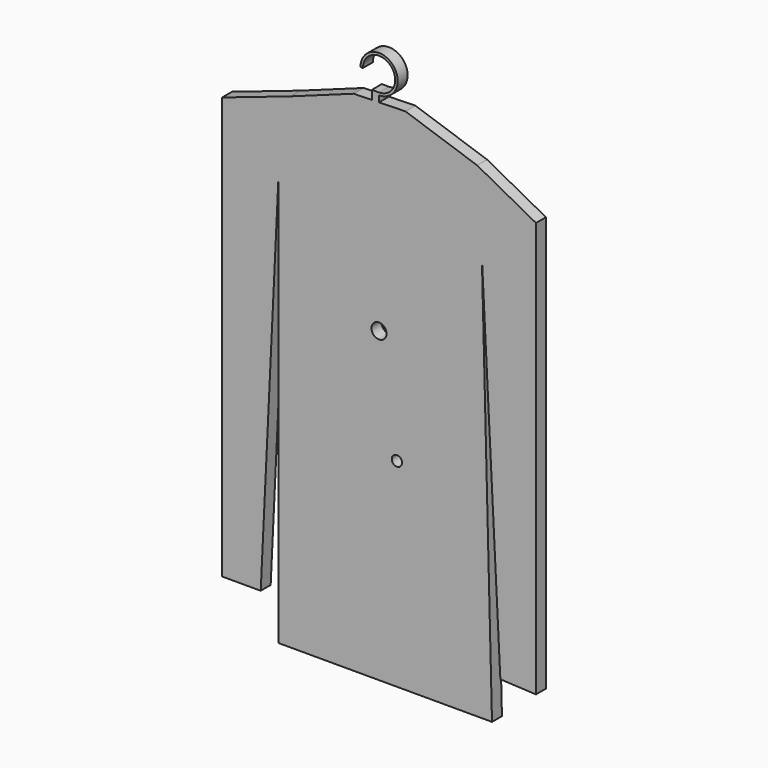
from build123d import *

# Parameters (mm, degrees)
F0_R     = 10.3520416824
F0_R_2   = 15.1016918028
F1_DEPTH = 12.5


with BuildPart() as f1:
    # F0 (on Front) → F1 (new body, symmetric)
    with BuildSketch(Plane.XZ):
        Polygon((-315.6363590755, 402.8576135222), (-315.6363590755, -445.1646387913), (-237.9194677537, -445.1646387913), (-202.4295538493, 294.5199684009), (-202.4295538493, -526.0605984591), (227.1852354976, -526.0605984591), (206.6384547892, 294.5199684009), (243.9962564237, -445.1646387913), (315.6363590755, -448.601916045), (315.6363590755, 386.046592596), (197.2990004611, 449.5548381291), (53.1655277069, 498.2233074495), (0, 496.8920787035), (-14.4139876592, 496.531162231), (-50.8757645807, 495.6181840727), (-178.146982003, 449.5548381291), align=None)
        with Locations((35.982593894, -126.2090504169)):
            Circle(F0_R, mode=Mode.SUBTRACT)
        with Locations((0, 92.1598300338)):
            Circle(F0_R_2, mode=Mode.SUBTRACT)
        with BuildLine():
            Line((-14.4139876592, 514.4077504381), (-14.4139876592, 496.531162231))
            Line((-14.4139876592, 496.531162231), (0, 496.8920787035))
            Line((0, 496.8920787035), (0, 509.4077504381))
            ThreePointArc((0, 509.4077504381), (26.5864663022, 573.3541076459), (-37.4994765184, 547.1058939281))
            Line((-37.4994765184, 547.1058939281), (-32.499546316, 547.0794747961))
            ThreePointArc((-32.499546316, 547.0794747961), (23.0416041286, 569.8279266848), (0, 514.4077504381))
            Line((0, 514.4077504381), (-14.4139876592, 514.4077504381))
        make_face()
    extrude(amount=F1_DEPTH, both=True)


solid = f1.part
